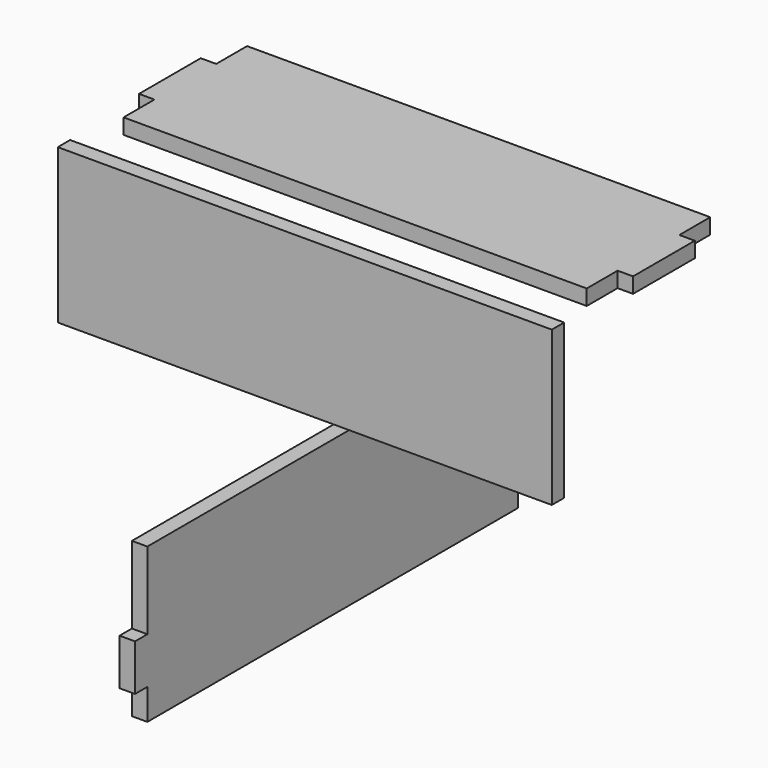
from build123d import *

# Parameters (mm, degrees)
F0_W     = 320
F0_H     = 100
F1_DEPTH = 10
F2_W     = 10
F2_H     = 50
F3_DEPTH = 10
F5_DEPTH = 10


# Not quite as in the source:
# - a feature names something its author has since deleted; it is built from what else it names


with BuildPart() as f1:
    # F0 (on Front) → F1 (new body)
    with BuildSketch(Plane.XZ):
        Rectangle(F0_W, F0_H)
    extrude(amount=F1_DEPTH)


with BuildPart() as f3:
    # F2 (on Top) → F3 (new body)
    with BuildSketch(Plane.XY):
        Polygon((-202.3773396015, 96.2469950318), (97.6226603985, 96.2469950318), (97.6226603985, 121.2469950318), (97.6226603985, 171.2469950318), (97.6226603985, 196.2469950318), (-202.3773396015, 196.2469950318), (-202.3773396015, 171.2469950318), (-202.3773396015, 121.2469950318), align=None)
        with Locations((-207.3773396015, 146.2469950318)):
            Rectangle(F2_W, F2_H)
        with Locations((102.6226603985, 146.2469950318)):
            Rectangle(F2_W, F2_H)
    extrude(amount=F3_DEPTH)


with BuildPart() as f5:
    # F4 (on Right) → F5 (new body)
    with BuildSketch(Plane.YZ):
        Polygon((-149.9543616176, -165.5762195587), (150.0456550453, -165.5762195587), (150.1001544525, -145.3023395036), (160.0456383824, -145.2841836565), (160.0456383824, -115.2841341545), (150.0456550453, -115.3023894922), (149.9546114852, -65.5762195587), (-149.9543616176, -65.5762195587), (-149.9543616176, -115.5762195587), (-159.9543616176, -115.5762195587), (-159.9543616176, -145.5762195587), (-149.9543616176, -145.5762195587), align=None)
    extrude(amount=F5_DEPTH)


solid = Compound([f1.part, f3.part, f5.part])
